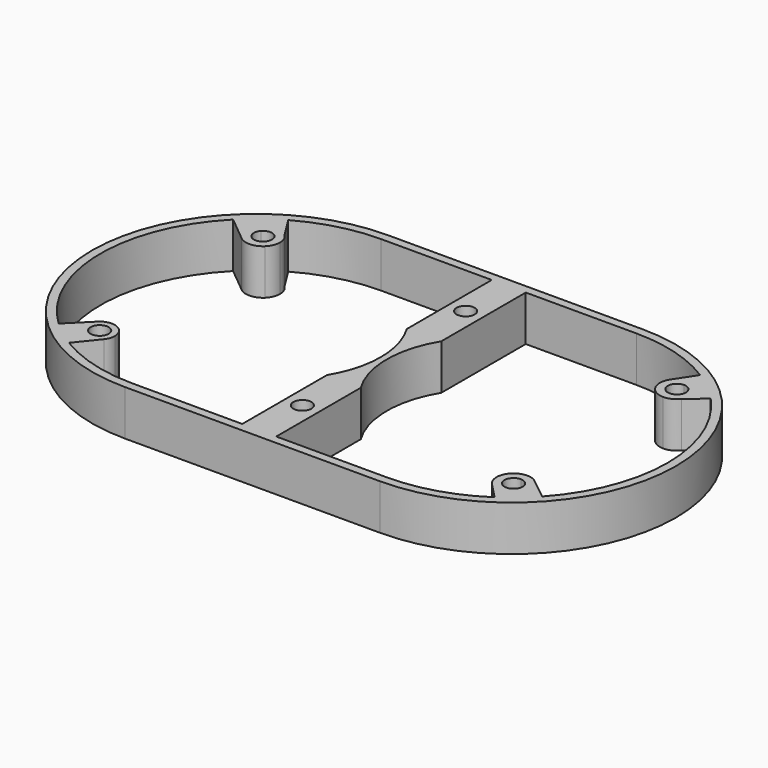
from build123d import *

# Parameters (mm, degrees)
F0_R     = 1.6
F1_DEPTH = 8


with BuildPart() as f1:
    # F0 (on Top) → F1 (new body)
    with BuildSketch(Plane.XY):
        with BuildLine():
            ThreePointArc((7.75, 8.769357237), (9.5785114413, 4.5384947039), (10.2033247314, -0.028042301))
            ThreePointArc((10.2033247314, -0.028042301), (9.5785114413, -4.5945793059), (7.75, -8.825441839))
            Line((7.75, -8.825441839), (7.75, -18.0000000146))
            ThreePointArc((7.75, -18.0000000146), (10.7499999927, -15), (13.75, -18))
            Line((13.75, -18), (13.75, -8.8741196746))
            ThreePointArc((13.75, -8.8741196746), (11.25, 0), (13.75, 8.8741196746))
            Line((13.75, 8.8741196746), (13.75, 18))
            ThreePointArc((13.75, 18), (10.75, 15), (7.75, 18))
            Line((7.75, 18), (7.75, 8.769357237))
        make_face()
        with BuildLine():
            Line((7.75, 27.5), (7.75, 18))
            ThreePointArc((7.75, 18), (10.75, 21), (13.75, 18))
            Line((13.75, 18), (13.75, 27.5))
            Line((13.75, 27.5), (7.75, 27.5))
        make_face()
        with BuildLine():
            ThreePointArc((13.75, 18), (10.75, 21), (7.75, 18))
            ThreePointArc((7.75, 18), (10.75, 15), (13.75, 18))
        make_face()
        with Locations((10.75, 18)):
            Circle(F0_R, mode=Mode.SUBTRACT)
        with BuildLine():
            ThreePointArc((13.75, -18), (10.7499999927, -15), (7.75, -18.0000000146))
            ThreePointArc((7.75, -18.0000000146), (10.7500000073, -21), (13.75, -18))
        make_face()
        with Locations((10.75, -18)):
            Circle(F0_R, mode=Mode.SUBTRACT)
        with BuildLine():
            ThreePointArc((13.75, -18), (10.7500000073, -21), (7.75, -18.0000000146))
            Line((7.75, -18.0000000146), (7.75, -27.5))
            Line((7.75, -27.5), (13.75, -27.5))
            Line((13.75, -27.5), (13.75, -18))
        make_face()
        with BuildLine():
            ThreePointArc((-25.2919277241, 23.9346233209), (-18.7517090297, 26.593722392), (-11.75, 27.5))
            Line((-11.75, 27.5), (-11.75, 29))
            ThreePointArc((-11.75, 29), (-40.75, 0), (-11.75, -29))
            Line((-11.75, -29), (-11.75, -27.5))
            ThreePointArc((-11.75, -27.5), (-19.1538130954, -26.4845908341), (-26.0108698504, -23.5133492108))
            ThreePointArc((-26.0108698504, -23.5133492108), (-27.4397291664, -22.5850038451), (-28.8083510414, -21.5699480701))
            ThreePointArc((-28.8083510414, -21.5699480701), (-29.7732335043, -20.7704851664), (-30.7006958236, -19.9278982284))
            ThreePointArc((-30.7006958236, -19.9278982284), (-39.2465788178, -0.4337664292), (-31.3198462511, 19.3202256122))
            ThreePointArc((-31.3198462511, 19.3202256122), (-30.0815714824, 20.4988655048), (-28.77245464, 21.5982878495))
            ThreePointArc((-28.77245464, 21.5982878495), (-27.0767734107, 22.8328714098), (-25.2919277241, 23.9346233209))
        make_face()
        Polygon((-11.75, 29), (-11.75, 27.5), (7.75, 27.5), (13.75, 27.5), (33.25, 27.5), (33.25, 29), align=None)
        Polygon((7.75, -27.5), (-11.75, -27.5), (-11.75, -29), (33.25, -29), (33.25, -27.5), (13.75, -27.5), align=None)
        with BuildLine():
            Line((-23.9181566023, 16.8211807336), (-22.9196159905, 15.8385184773))
            ThreePointArc((-22.9196159905, 15.8385184773), (-22.2394609196, 16.8255111811), (-22, 18))
            ThreePointArc((-22, 18), (-22.2419209631, 19.180254221), (-22.9286666841, 20.1701562834))
            ThreePointArc((-22.9286666841, 20.1701562834), (-25.0876469222, 20.9987193962), (-27.1945482113, 20.0454725978))
            Line((-27.1945482113, 20.0454725978), (-26.1960075994, 19.0628103416))
            ThreePointArc((-26.1960075994, 19.0628103416), (-24.4314985308, 19.4955955601), (-23.4, 18))
            ThreePointArc((-23.4, 18), (-23.5352560913, 17.3561636218), (-23.9181566023, 16.8211807336))
        make_face()
        with BuildLine():
            ThreePointArc((-27.0590321397, 15.818168969), (-24.9852520778, 15.0000362504), (-22.9196159905, 15.8385184773))
            Line((-22.9196159905, 15.8385184773), (-23.9181566023, 16.8211807336))
            ThreePointArc((-23.9181566023, 16.8211807336), (-26.122267433, 16.8595984002), (-26.1960075994, 19.0628103416))
            Line((-26.1960075994, 19.0628103416), (-27.1945482113, 20.0454725978))
            ThreePointArc((-27.1945482113, 20.0454725978), (-27.9984596784, 17.9038773857), (-27.0590321397, 15.818168969))
        make_face()
        with BuildLine():
            Line((-22.9286666841, 20.1701562834), (-25.2919277241, 23.9346233209))
            ThreePointArc((-25.2919277241, 23.9346233209), (-27.0767734107, 22.8328714098), (-28.77245464, 21.5982878495))
            Line((-28.77245464, 21.5982878495), (-27.1945482113, 20.0454725978))
            ThreePointArc((-27.1945482113, 20.0454725978), (-25.0876469222, 20.9987193962), (-22.9286666841, 20.1701562834))
        make_face()
        with BuildLine():
            ThreePointArc((-22.3292838603, -18), (-22.5488627131, -16.9395045028), (-23.1714929463, -16.053390986))
            Line((-23.1714929463, -16.053390986), (-23.9378571629, -16.8033995681))
            ThreePointArc((-23.9378571629, -16.8033995681), (-23.5406459409, -17.3440383164), (-23.4, -18))
            ThreePointArc((-23.4, -18), (-24.4480811477, -19.5017941205), (-26.2192319756, -19.0360856093))
            Line((-26.2192319756, -19.0360856093), (-26.9855961921, -19.7860941914))
            ThreePointArc((-26.9855961921, -19.7860941914), (-24.9271170835, -20.6697214797), (-22.9199137797, -19.6751017924))
            ThreePointArc((-22.9199137797, -19.6751017924), (-22.4812657406, -18.8880892011), (-22.3292838603, -18))
        make_face()
        with BuildLine():
            Line((-23.9378571629, -16.8033995681), (-23.1714929463, -16.053390986))
            ThreePointArc((-23.1714929463, -16.053390986), (-25.0424895986, -15.3296218746), (-26.8895125058, -16.1125500829))
            ThreePointArc((-26.8895125058, -16.1125500829), (-27.6698030703, -17.9301697453), (-26.9855961921, -19.7860941914))
            Line((-26.9855961921, -19.7860941914), (-26.2192319756, -19.0360856093))
            ThreePointArc((-26.2192319756, -19.0360856093), (-26.1191027607, -16.8564926712), (-23.9378571629, -16.8033995681))
        make_face()
        with BuildLine():
            ThreePointArc((-28.8083510414, -21.5699480701), (-27.4397291664, -22.5850038451), (-26.0108698504, -23.5133492108))
            Line((-26.0108698504, -23.5133492108), (-22.9199137797, -19.6751017924))
            ThreePointArc((-22.9199137797, -19.6751017924), (-24.9271170835, -20.6697214797), (-26.9855961921, -19.7860941914))
            Line((-26.9855961921, -19.7860941914), (-28.8083510414, -21.5699480701))
        make_face()
        with BuildLine():
            Line((-31.3198462511, 19.3202256122), (-27.0590321397, 15.818168969))
            ThreePointArc((-27.0590321397, 15.818168969), (-27.9984596784, 17.9038773857), (-27.1945482113, 20.0454725978))
            Line((-27.1945482113, 20.0454725978), (-28.77245464, 21.5982878495))
            ThreePointArc((-28.77245464, 21.5982878495), (-30.0815714824, 20.4988655048), (-31.3198462511, 19.3202256122))
        make_face()
        with BuildLine():
            ThreePointArc((33.25, -29), (62.25, 0), (33.25, 29))
            Line((33.25, 29), (33.25, 27.5))
            ThreePointArc((33.25, 27.5), (40.8605006229, 26.4259395343), (47.8765184935, 23.2876567468))
            ThreePointArc((47.8765184935, 23.2876567468), (50.7935969105, 21.177162403), (53.4099454165, 18.7036520713))
            ThreePointArc((53.4099454165, 18.7036520713), (60.7498923776, 0.0769364868), (53.514283477, -18.5905571505))
            ThreePointArc((53.514283477, -18.5905571505), (51.1559396917, -20.8716871325), (48.5427019981, -22.8557053183))
            ThreePointArc((48.5427019981, -22.8557053183), (41.2411858865, -26.3133226356), (33.25, -27.5))
            Line((33.25, -27.5), (33.25, -29))
        make_face()
        with BuildLine():
            ThreePointArc((-26.9855961921, -19.7860941914), (-27.6698030703, -17.9301697453), (-26.8895125058, -16.1125500829))
            Line((-26.8895125058, -16.1125500829), (-30.7006958236, -19.9278982284))
            ThreePointArc((-30.7006958236, -19.9278982284), (-29.7732335043, -20.7704851664), (-28.8083510414, -21.5699480701))
            Line((-28.8083510414, -21.5699480701), (-26.9855961921, -19.7860941914))
        make_face()
        with BuildLine():
            ThreePointArc((53.4099454165, 18.7036520713), (50.7935969105, 21.177162403), (47.8765184935, 23.2876567468))
            Line((47.8765184935, 23.2876567468), (45.4902157392, 19.6434667518))
            ThreePointArc((45.4902157392, 19.6434667518), (48.8575101217, 20.8748350198), (51, 18))
            ThreePointArc((51, 18), (50.8256587545, 16.9922040865), (50.3228982644, 16.1015417695))
            Line((50.3228982644, 16.1015417695), (53.4099454165, 18.7036520713))
        make_face()
        with BuildLine():
            Line((46.1222517122, -20.3396712093), (48.5427019981, -22.8557053183))
            ThreePointArc((48.5427019981, -22.8557053183), (51.1559396917, -20.8716871325), (53.514283477, -18.5905571505))
            Line((53.514283477, -18.5905571505), (50.1028595569, -15.8603781447))
            ThreePointArc((50.1028595569, -15.8603781447), (50.7666386348, -16.8399523007), (51, -18))
            ThreePointArc((51, -18), (49.2974504107, -20.7049255871), (46.1222517122, -20.3396712093))
        make_face()
        with BuildLine():
            ThreePointArc((51, 18), (48.8575101217, 20.8748350198), (45.4902157392, 19.6434667518))
            ThreePointArc((45.4902157392, 19.6434667518), (45.3608334407, 16.5735358847), (48, 15))
            ThreePointArc((48, 15), (49.2854231421, 15.2893382089), (50.3228982644, 16.1015417695))
            ThreePointArc((50.3228982644, 16.1015417695), (50.8256587545, 16.9922040865), (51, 18))
        make_face()
        with BuildLine():
            ThreePointArc((49.6, 18), (49.1313708499, 16.8686291501), (48, 16.4))
            ThreePointArc((48, 16.4), (46.4, 18), (48, 19.6))
            ThreePointArc((48, 19.6), (49.1313708499, 19.1313708499), (49.6, 18))
        make_face(mode=Mode.SUBTRACT)
        with BuildLine():
            Line((45.5893930702, -19.7857699264), (46.1222517122, -20.3396712093))
            ThreePointArc((46.1222517122, -20.3396712093), (49.2974504107, -20.7049255871), (51, -18))
            ThreePointArc((51, -18), (50.7666386348, -16.8399523007), (50.1028595569, -15.8603781447))
            Line((50.1028595569, -15.8603781447), (49.6267696131, -15.4793610679))
            ThreePointArc((49.6267696131, -15.4793610679), (48.8479632079, -15.1223345576), (48, -15))
            ThreePointArc((48, -15), (45.3206988057, -16.6504278047), (45.5893930702, -19.7857699264))
        make_face()
        with BuildLine():
            ThreePointArc((49.6, -18), (46.8686291501, -19.1313708499), (48, -16.4))
            ThreePointArc((48, -16.4), (49.1313708499, -16.8686291501), (49.6, -18))
        make_face(mode=Mode.SUBTRACT)
    extrude(amount=F1_DEPTH)


solid = f1.part
